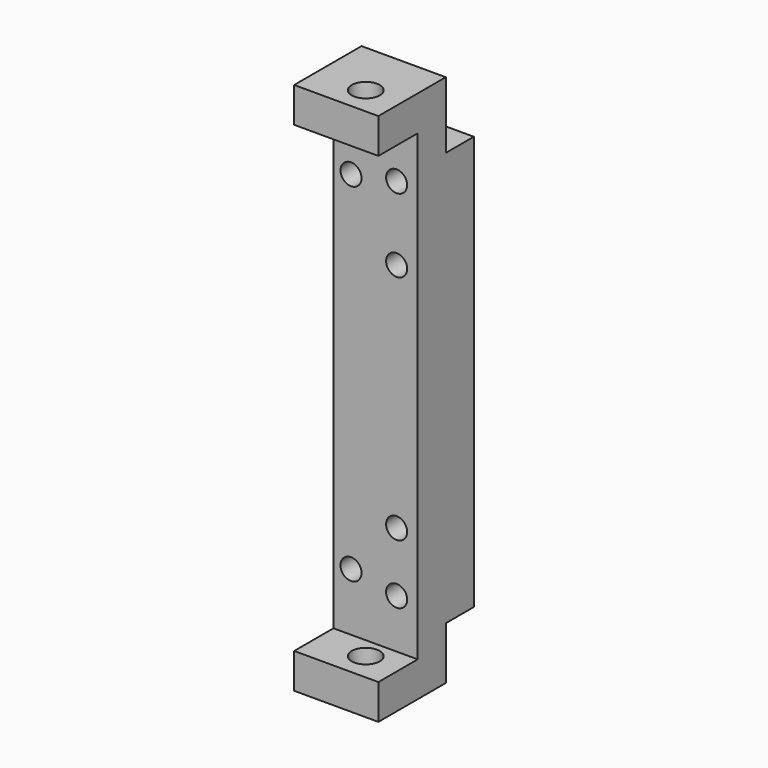
from build123d import *

# Parameters (mm, degrees)
F1_DEPTH  = 12
F2_W      = 6.02
F2_H      = 5
F3_DEPTH  = 76
F4_R      = 1.5
F5_DEPTH  = 25
F6_R      = 1.5
F7_DEPTH  = 25
F8_W      = 12
F8_H      = 5
F9_DEPTH  = 7
F10_R     = 2
F11_DEPTH = 76
F12_W     = 5.98
F12_H     = 9.5
F12_H_2   = 7.5
F13_DEPTH = 5
F14_R     = 1.5
F15_DEPTH = 25


# Not quite as in the source:
# - a feature names something its author has since deleted; it is built from what else it names


with BuildPart() as f1:
    # F0 (on Right) → F1 (new body)
    with BuildSketch(Plane.YZ):
        Polygon((13.5, 40.5), (-3.5, 40.5), (-3.5, 35.5), (3.5, 35.5), (3.5, -35.5), (13.5, -35.5), align=None)
    extrude(amount=F1_DEPTH)

    # F2 (on face) → F3 (cut)
    with BuildSketch(Plane.XY.offset(40.5)):
        with Locations((3.01, 11)):
            Rectangle(F2_W, F2_H)
    extrude(amount=-F3_DEPTH, mode=Mode.SUBTRACT)

    # F4 (on face) → F5 (cut)
    with BuildSketch(Plane(origin=(0, 13.5, 0), x_dir=(-1, 0, 0), z_dir=(0, 1, 0))):
        with Locations((-9, 28.5)):
            Circle(F4_R)
        with Locations((-9, -23.5)):
            Circle(F4_R)
    extrude(amount=-F5_DEPTH, mode=Mode.SUBTRACT)

    # F6 (on face) → F7 (cut)
    with BuildSketch(Plane(origin=(0, 8.5, 0), x_dir=(-1, 0, 0), z_dir=(0, 1, 0))):
        with Locations((-2.5, -22.265)):
            Circle(F6_R)
        with Locations((-2.5, 27.265)):
            Circle(F6_R)
    extrude(amount=-F7_DEPTH, mode=Mode.SUBTRACT)

    # F8 (on face) → F9 (join)
    with BuildSketch(Plane.XZ.offset(-3.5)):
        with Locations((6, -33)):
            Rectangle(F8_W, F8_H)
    extrude(amount=F9_DEPTH)

    # F10 (on face) → F11 (cut)
    with BuildSketch(Plane.XY.offset(40.5)):
        with Locations((7, 0.5)):
            Circle(F10_R)
    extrude(amount=-F11_DEPTH, mode=Mode.SUBTRACT)

    # F12 (on face) → F13 (cut)
    with BuildSketch(Plane(origin=(0, 13.5, 0), x_dir=(-1, 0, 0), z_dir=(0, 1, 0))):
        with Locations((-9.01, 35.75)):
            Rectangle(F12_W, F12_H)
        with Locations((-9.01, -31.75)):
            Rectangle(F12_W, F12_H_2)
    extrude(amount=-F13_DEPTH, mode=Mode.SUBTRACT)

    # F14 (on face) → F15 (cut)
    with BuildSketch(Plane(origin=(0, 13.5, 0), x_dir=(-1, 0, 0), z_dir=(0, 1, 0))):
        with Locations((-9, -15)):
            Circle(F14_R)
        with Locations((-9, 18)):
            Circle(F14_R)
    extrude(amount=-F15_DEPTH, mode=Mode.SUBTRACT)


solid = f1.part
